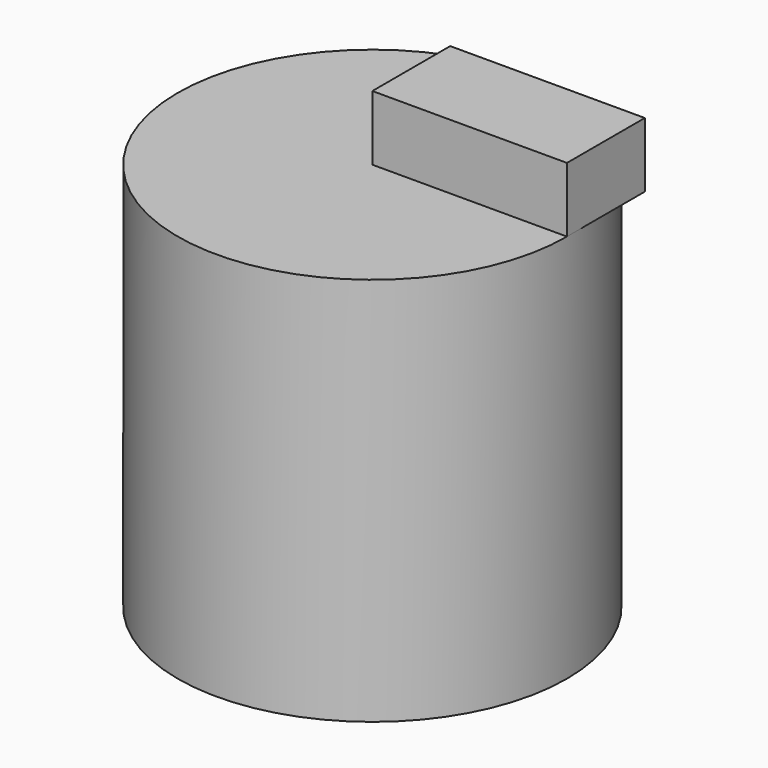
from build123d import *

# Parameters (mm, degrees)
F2_DEPTH = 25.4
F0_R     = 76.2
F3_DEPTH = 152.4
F4_DEPTH = 152.4


# Not quite as in the source:
# - an extrude ends at something that could not be found from the text; its depth is read off the source's solid


with BuildPart() as f2:
    # F1 (on Top) → F2 (new body)
    with BuildSketch(Plane.XY):
        with BuildLine():
            Line((0, 19.05), (0, 0))
            Line((0, 0), (19.05, 0))
            ThreePointArc((19.05, 0), (5.5796158184, 5.5796158184), (0, 19.05))
        make_face()
        with BuildLine():
            ThreePointArc((0, 19.05), (5.5796158184, 5.5796158184), (19.05, 0))
            Line((19.05, 0), (57.15, 0))
            ThreePointArc((57.15, 0), (70.6203841816, 5.5796158184), (76.2, 19.05))
            ThreePointArc((76.2, 19.05), (70.6203841816, 32.5203841816), (57.15, 38.1))
            Line((57.15, 38.1), (19.05, 38.1))
            ThreePointArc((19.05, 38.1), (5.5796158184, 32.5203841816), (0, 19.05))
        make_face()
        with BuildLine():
            Line((0, 38.1), (0, 19.05))
            ThreePointArc((0, 19.05), (5.5796158184, 32.5203841816), (19.05, 38.1))
            Line((19.05, 38.1), (0, 38.1))
        make_face()
        with BuildLine():
            ThreePointArc((76.2, 19.05), (70.6203841816, 5.5796158184), (57.15, 0))
            Line((57.15, 0), (76.2, 0))
            Line((76.2, 0), (76.2, 19.05))
        make_face()
        with BuildLine():
            ThreePointArc((57.15, 38.1), (70.6203841816, 32.5203841816), (76.2, 19.05))
            Line((76.2, 19.05), (76.2, 38.1))
            Line((76.2, 38.1), (57.15, 38.1))
        make_face()
    extrude(amount=F2_DEPTH)

    # F0 (on Top) → F3 (join, through all)
    with BuildSketch(Plane.XY):
        Circle(F0_R)
    extrude(amount=-F3_DEPTH)

    # F0 (on Top) → F4 (join)
    with BuildSketch(Plane.XY):
        Circle(F0_R)
    extrude(amount=-F4_DEPTH)


solid = f2.part
